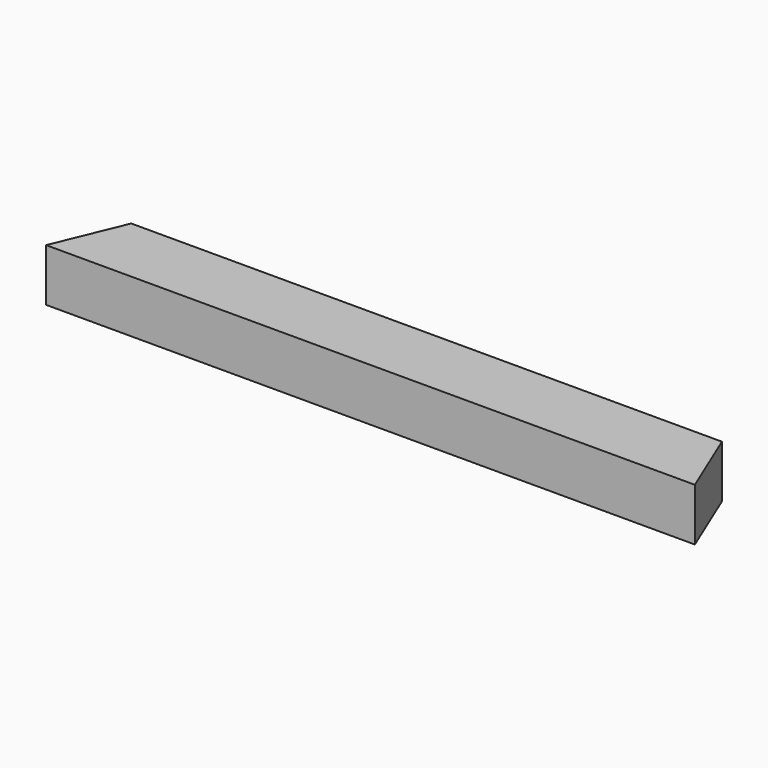
from build123d import *

# Parameters (mm, degrees)
F0_W     = 203.2
F0_H     = 152.4
F1_DEPTH = 939.8
F3_DEPTH = 152.401


# Not quite as in the source:
# - a pattern or mirror of a feature is missing from the dataset's text; its kind, count and spacing are read off the source's solid


with BuildPart() as f1:
    # F0 (on Right) → F1 (new body, symmetric)
    with BuildSketch(Plane.YZ):
        Rectangle(F0_W, F0_H)
    extrude(amount=F1_DEPTH, both=True)

    # F2 (on face) → F3 (cut, through all)
    with BuildSketch(Plane.XY.offset(76.2)):
        Polygon((-939.8, 101.6), (-939.8, -101.6), (-855.6318041258, 101.6), align=None)
    f3 = extrude(amount=-F3_DEPTH, mode=Mode.SUBTRACT)

    # F3_copies: F3 across plane
    add(f3.mirror(Plane(origin=(0, 0, 0), x_dir=(0, 0, 1), z_dir=(1, 0, 0))), mode=Mode.SUBTRACT)


solid = f1.part
